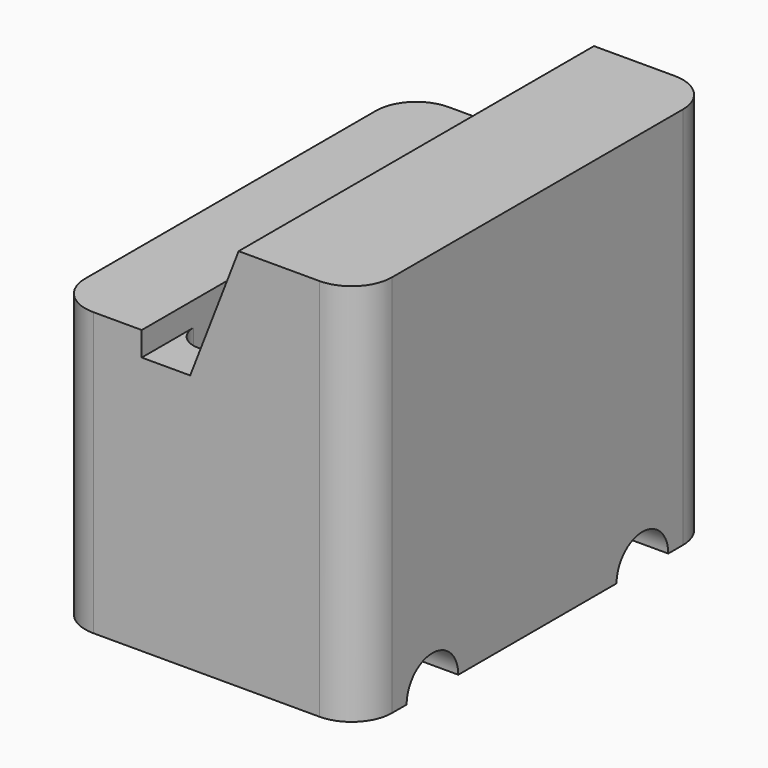
from build123d import *

# Parameters (mm, degrees)
F1_DEPTH = 55
F3_DEPTH = 32.001
F4_R     = 5
F5_R     = 5
F7_DEPTH = 20
F9_DEPTH = 6


# Not quite as in the source:
# - a feature names something its author has since deleted; it is built from what else it names


with BuildPart() as f1:
    # F0 (on Front) → F1 (new body)
    with BuildSketch(Plane.XZ):
        Polygon((0, 35), (0, 0), (38, 0), (38, 47.5), (23, 47.5), (17, 32), (11, 32), (11, 35), align=None)
    extrude(amount=F1_DEPTH)

    # F2 (on face) → F3 (cut, through all)
    with BuildSketch(Plane.XY.offset(32)):
        with BuildLine():
            ThreePointArc((14, -5), (11.8786796564, -5.8786796564), (11, -8))
            Line((11, -8), (11, -14.5))
            ThreePointArc((11, -14.5), (11.8786796564, -16.6213203436), (14, -17.5))
            ThreePointArc((14, -17.5), (16.1213203436, -16.6213203436), (17, -14.5))
            Line((17, -14.5), (17, -8))
            ThreePointArc((17, -8), (16.1213203436, -5.8786796564), (14, -5))
        make_face()
        with BuildLine():
            ThreePointArc((14, -37.5), (11.8786796564, -38.3786796564), (11, -40.5))
            Line((11, -40.5), (11, -47))
            ThreePointArc((11, -47), (11.8786796564, -49.1213203436), (14, -50))
            ThreePointArc((14, -50), (16.1213203436, -49.1213203436), (17, -47))
            Line((17, -47), (17, -40.5))
            ThreePointArc((17, -40.5), (16.1213203436, -38.3786796564), (14, -37.5))
        make_face()
    extrude(amount=-F3_DEPTH, mode=Mode.SUBTRACT)

    # F4
    f4_edges = [f1.edges().sort_by_distance(p)[0] for p in [
        (38, -55, 23.75),
        (38, 0, 23.75),
    ]]
    fillet(f4_edges, radius=F4_R)

    # F5
    f5_edges = [f1.edges().sort_by_distance(p)[0] for p in [
        (0, 0, 17.5),
        (0, -55, 17.5),
    ]]
    fillet(f5_edges, radius=F5_R)

    # F6 (on face) → F7 (cut)
    with BuildSketch(Plane(origin=(0, 0, 0), x_dir=(1, 0, 0), z_dir=(0, 0, -1))):
        with BuildLine():
            Line((27, 52), (7, 52))
            ThreePointArc((7, 52), (3.4644660941, 50.5355339059), (2, 47))
            Line((2, 47), (2, 8))
            ThreePointArc((2, 8), (3.4644660941, 4.4644660941), (7, 3))
            Line((7, 3), (27, 3))
            ThreePointArc((27, 3), (30.5355339059, 4.4644660941), (32, 8))
            Line((32, 8), (32, 47))
            ThreePointArc((32, 47), (30.5355339059, 50.5355339059), (27, 52))
        make_face()
        with BuildLine():
            ThreePointArc((17, 8), (14, 5), (11, 8))
            Line((11, 8), (11, 14.5))
            ThreePointArc((11, 14.5), (14, 17.5), (17, 14.5))
            Line((17, 14.5), (17, 8))
        make_face(mode=Mode.SUBTRACT)
        with BuildLine():
            Line((17, 47), (17, 40.5))
            ThreePointArc((17, 40.5), (14, 37.5), (11, 40.5))
            Line((11, 40.5), (11, 47))
            ThreePointArc((11, 47), (14, 50), (17, 47))
        make_face(mode=Mode.SUBTRACT)
    extrude(amount=-F7_DEPTH, mode=Mode.SUBTRACT)

    # F8 (on face) → F9 (cut)
    with BuildSketch(Plane.YZ.offset(38)):
        with BuildLine():
            Line((-47.75, 0), (-39.75, 0))
            ThreePointArc((-39.75, 0), (-43.75, 4), (-47.75, 0))
        make_face()
        with BuildLine():
            ThreePointArc((-7.25, 0), (-11.25, 4), (-15.25, 0))
            Line((-15.25, 0), (-7.25, 0))
        make_face()
    extrude(amount=-F9_DEPTH, mode=Mode.SUBTRACT)


solid = f1.part
